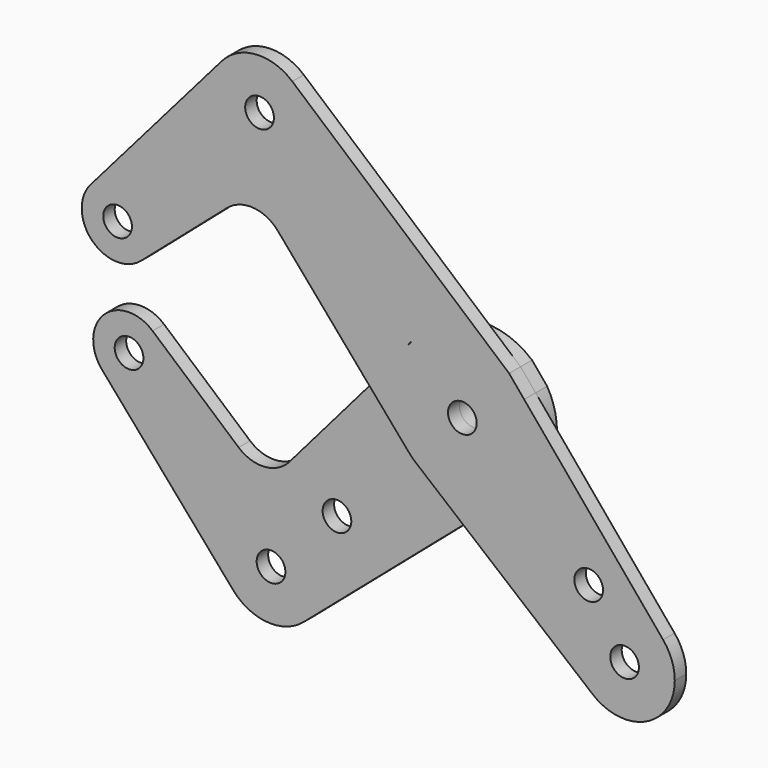
from build123d import *

# Parameters (mm, degrees)
F0_R     = 3.175
F0_R_2   = 3.9751
F1_DEPTH = 3.175
F2_DEPTH = 3.175


# Not quite as in the source:
# - a feature names something its author has since deleted; it is built from what else it names


with BuildPart() as f1:
    # F0 (on Front) → F1 (new body)
    with BuildSketch(Plane.XZ):
        with BuildLine():
            ThreePointArc((-71.1347575644, 7.4711561347), (-69.1121208226, 10.1727039932), (-68.3946770291, 13.4703841816))
            ThreePointArc((-68.3946770291, 13.4703841816), (-73.5586383483, 20.9075469092), (-82.331405076, 18.6678036462))
            ThreePointArc((-82.331405076, 18.6678036462), (-81.9448371048, 7.8577241059), (-71.1347575644, 7.4711561347))
        make_face()
        with Locations((-76.3321770291, 13.4703841816)):
            Circle(F0_R, mode=Mode.SUBTRACT)
        with BuildLine():
            ThreePointArc((-82.331405076, 18.6678036462), (-73.5586383483, 20.9075469092), (-68.3946770291, 13.4703841816))
            ThreePointArc((-68.3946770291, 13.4703841816), (-69.1121208226, 10.1727039932), (-71.1347575644, 7.4711561347))
            Line((-71.1347575644, 7.4711561347), (-52.0843267669, 23.9754595323))
            ThreePointArc((-52.0843267669, 23.9754595323), (-46.2965222838, 25.8954961667), (-40.8511612346, 23.1508168672))
            Line((-40.8511612346, 23.1508168672), (-20.9164773453, -0.0263913939))
            Line((-20.9164773453, -0.0263913939), (-12.7650204358, 9.4376839465))
            ThreePointArc((-12.7650204358, 9.4376839465), (-12.0284255483, 10.3601449714), (-11.2253201513, 11.2253201513))
            ThreePointArc((-11.2253201513, 11.2253201513), (-0.5957321126, 15.8638182116), (10.3518054047, 12.0356034274))
            Line((10.3518054047, 12.0356034274), (-37.655016822, 53.3262030046))
            ThreePointArc((-37.655016822, 53.3262030046), (-34.8014845049, 49.5361241819), (-33.7887806053, 44.9012806053))
            ThreePointArc((-33.7887806053, 44.9012806053), (-48.7842347585, 34.4892527868), (-53.300199871, 52.1776678558))
            Line((-53.300199871, 52.1776678558), (-82.331405076, 18.6678036462))
        make_face()
        with BuildLine():
            ThreePointArc((-37.655016822, 53.3262030046), (-45.7148756595, 55.9839571475), (-53.300199871, 52.1776678558))
            ThreePointArc((-53.300199871, 52.1776678558), (-48.7842347585, 34.4892527868), (-33.7887806053, 44.9012806053))
            ThreePointArc((-33.7887806053, 44.9012806053), (-34.8014845049, 49.5361241819), (-37.655016822, 53.3262030046))
        make_face()
        with Locations((-44.9012806053, 44.9012806053)):
            Circle(F0_R, mode=Mode.SUBTRACT)
        with BuildLine():
            Line((13.6886557503, 8.0396721793), (10.3518054047, 12.0356034274))
            ThreePointArc((10.3518054047, 12.0356034274), (-0.5957321126, 15.8638182116), (-11.2253201513, 11.2253201513))
            Line((-11.2253201513, 11.2253201513), (-12.7650204358, 9.4376839465))
            ThreePointArc((-12.7650204358, 9.4376839465), (-15.8642273117, -0.5847365245), (-12.0356034274, -10.3518054047))
            ThreePointArc((-12.0356034274, -10.3518054047), (-11.1192092809, -11.3304373246), (-10.1235074968, -12.2282550252))
            ThreePointArc((-10.1235074968, -12.2282550252), (0.1493608834, -15.8742973491), (10.3518055584, -12.0356032953))
            ThreePointArc((10.3518055584, -12.0356032953), (14.4282801858, -6.6212050173), (15.875, 0))
            ThreePointArc((15.875, 0), (15.3186656572, 4.1658261464), (13.6886557503, 8.0396721793))
        make_face()
        Circle(F0_R_2, mode=Mode.SUBTRACT)
        with BuildLine():
            Line((-12.7650204358, 9.4376839465), (-20.9164773453, -0.0263913939))
            Line((-20.9164773453, -0.0263913939), (-12.0356034274, -10.3518054047))
            ThreePointArc((-12.0356034274, -10.3518054047), (-15.8642273117, -0.5847365245), (-12.7650204358, 9.4376839465))
        make_face()
        with BuildLine():
            Line((44.4506274521, -28.7982771588), (13.6886557503, 8.0396721793))
            ThreePointArc((13.6886557503, 8.0396721793), (15.3186656572, 4.1658261464), (15.875, 0))
            ThreePointArc((15.875, 0), (14.4282801858, -6.6212050173), (10.3518055584, -12.0356032953))
            Line((10.3518055584, -12.0356032953), (0.1954344954, -20.7710836138))
            Line((0.1954344954, -20.7710836138), (28.8345692365, -44.4808030019))
            ThreePointArc((28.8345692365, -44.4808030019), (28.0466309813, -28.0800052132), (44.4506274521, -28.7982771588))
        make_face()
        with Locations((27.9745180668, -23.4843900063)):
            Circle(F0_R, mode=Mode.SUBTRACT)
        with BuildLine():
            ThreePointArc((47.0335244843, -35.9210244843), (46.3678629828, -32.132723858), (44.4506274521, -28.7982771588))
            ThreePointArc((44.4506274521, -28.7982771588), (28.0466309813, -28.0800052132), (28.8345692365, -44.4808030019))
            ThreePointArc((28.8345692365, -44.4808030019), (40.650687385, -45.9767663811), (47.0335244843, -35.9210244843))
        make_face()
        with Locations((35.9210244843, -35.9210244843)):
            Circle(F0_R, mode=Mode.SUBTRACT)
        with BuildLine():
            ThreePointArc((10.3518055584, -12.0356032953), (0.1493608834, -15.8742973491), (-10.1235074968, -12.2282550252))
            Line((-10.1235074968, -12.2282550252), (0.1954344954, -20.7710836138))
            Line((0.1954344954, -20.7710836138), (10.3518055584, -12.0356032953))
        make_face()
        Circle(F0_R_2)
        Circle(F0_R, mode=Mode.SUBTRACT)
    extrude(amount=F1_DEPTH)


with BuildPart() as f2:
    # F0 (on Front) → F2 (new body)
    with BuildSketch(Plane.XZ):
        with BuildLine():
            ThreePointArc((-68.3946770291, -13.4703841816), (-69.1121208226, -10.1727039932), (-71.1347575644, -7.4711561347))
            ThreePointArc((-71.1347575644, -7.4711561347), (-81.9448371048, -7.8577241059), (-82.331405076, -18.6678036462))
            ThreePointArc((-82.331405076, -18.6678036462), (-73.5586383483, -20.9075469092), (-68.3946770291, -13.4703841816))
        make_face()
        with Locations((-76.3321770291, -13.4703841816)):
            Circle(F0_R, mode=Mode.SUBTRACT)
        with BuildLine():
            Line((-12.0356034274, -10.3518054047), (-20.9164773453, -0.0263913939))
            Line((-20.9164773453, -0.0263913939), (-40.8447372902, -23.1636729395))
            ThreePointArc((-40.8447372902, -23.1636729395), (-46.2892514984, -25.9043770281), (-52.0743081406, -23.9841391495))
            Line((-52.0743081406, -23.9841391495), (-71.1347575644, -7.4711561347))
            ThreePointArc((-71.1347575644, -7.4711561347), (-69.1121208226, -10.1727039932), (-68.3946770291, -13.4703841816))
            ThreePointArc((-68.3946770291, -13.4703841816), (-73.5586383483, -20.9075469092), (-82.331405076, -18.6678036462))
            Line((-82.331405076, -18.6678036462), (-53.300199871, -52.1776678558))
            ThreePointArc((-53.300199871, -52.1776678558), (-48.7842347585, -34.4892527868), (-33.7887806053, -44.9012806053))
            ThreePointArc((-33.7887806053, -44.9012806053), (-34.8014845049, -49.5361241819), (-37.655016822, -53.3262030046))
            Line((-37.655016822, -53.3262030046), (0.1954344954, -20.7710836138))
            Line((0.1954344954, -20.7710836138), (-10.1235074968, -12.2282550252))
            ThreePointArc((-10.1235074968, -12.2282550252), (-11.1192092809, -11.3304373246), (-12.0356034274, -10.3518054047))
        make_face()
        with Locations((-30.2993841525, -30.2993841525)):
            Circle(F0_R, mode=Mode.SUBTRACT)
        with BuildLine():
            ThreePointArc((-53.300199871, -52.1776678558), (-45.7148756595, -55.9839571475), (-37.655016822, -53.3262030046))
            ThreePointArc((-37.655016822, -53.3262030046), (-34.8014845049, -49.5361241819), (-33.7887806053, -44.9012806053))
            ThreePointArc((-33.7887806053, -44.9012806053), (-48.7842347585, -34.4892527868), (-53.300199871, -52.1776678558))
        make_face()
        with Locations((-44.9012806053, -44.9012806053)):
            Circle(F0_R, mode=Mode.SUBTRACT)
        with BuildLine():
            ThreePointArc((10.3518055584, -12.0356032953), (0.1493608834, -15.8742973491), (-10.1235074968, -12.2282550252))
            Line((-10.1235074968, -12.2282550252), (0.1954344954, -20.7710836138))
            Line((0.1954344954, -20.7710836138), (10.3518055584, -12.0356032953))
        make_face()
        with BuildLine():
            Line((-12.7650204358, 9.4376839465), (-20.9164773453, -0.0263913939))
            Line((-20.9164773453, -0.0263913939), (-12.0356034274, -10.3518054047))
            ThreePointArc((-12.0356034274, -10.3518054047), (-15.8642273117, -0.5847365245), (-12.7650204358, 9.4376839465))
        make_face()
        with BuildLine():
            Line((13.6886557503, 8.0396721793), (10.3518054047, 12.0356034274))
            ThreePointArc((10.3518054047, 12.0356034274), (-0.5957321126, 15.8638182116), (-11.2253201513, 11.2253201513))
            Line((-11.2253201513, 11.2253201513), (-12.7650204358, 9.4376839465))
            ThreePointArc((-12.7650204358, 9.4376839465), (-15.8642273117, -0.5847365245), (-12.0356034274, -10.3518054047))
            ThreePointArc((-12.0356034274, -10.3518054047), (-11.1192092809, -11.3304373246), (-10.1235074968, -12.2282550252))
            ThreePointArc((-10.1235074968, -12.2282550252), (0.1493608834, -15.8742973491), (10.3518055584, -12.0356032953))
            ThreePointArc((10.3518055584, -12.0356032953), (14.4282801858, -6.6212050173), (15.875, 0))
            ThreePointArc((15.875, 0), (15.3186656572, 4.1658261464), (13.6886557503, 8.0396721793))
        make_face()
        Circle(F0_R_2, mode=Mode.SUBTRACT)
        Circle(F0_R_2)
        Circle(F0_R, mode=Mode.SUBTRACT)
    extrude(amount=-F2_DEPTH)


solid = Compound([f1.part, f2.part])
